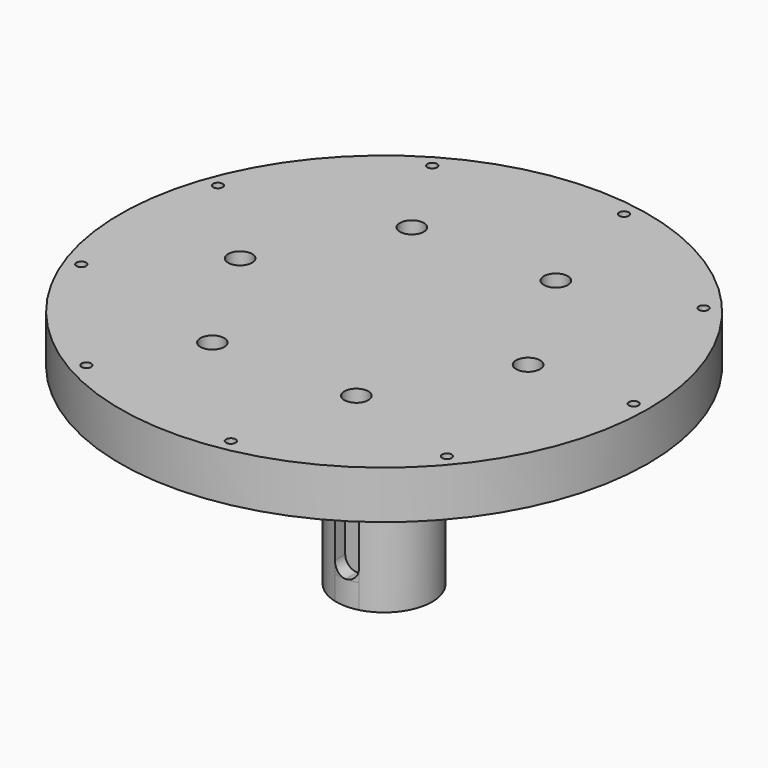
from build123d import *

# Parameters (mm, degrees)
F0_R         = 55
F0_R_2       = 1
F0_R_3       = 2.5
F0_R_4       = 10
F1_DEPTH     = 50
F1_FACE_R    = 55
F1_FACE_R_2  = 1
F1_FACE_R_3  = 2.5
F2_DEPTH     = 40
F3_R         = 7.5
F3_R_2       = 2.5
F4_DEPTH     = 5
F6_DEPTH     = 25
F7_DEPTH     = 5
F8_T4_DEPTH  = 15.1824583655
F8_S5_R      = 10
F8_T6_DEPTH  = 9
F8_T10_DEPTH = 15.1824583655
F8_S11_R     = 10
F8_T12_DEPTH = 9
F8_T16_DEPTH = 15.1824583655
F8_S17_R     = 10
F8_T18_DEPTH = 9
F8_T22_DEPTH = 15.1824583655
F8_S23_R     = 10
F8_T24_DEPTH = 9


# Not quite as in the source:
# - a fillet or chamfer that OpenCascade refuses, or shapes differently, is made with other operations: its cross-section is extruded or revolved along the edge and cut away or added


with BuildPart() as f1:
    # F0 (on Top) → F1 (new body)
    with BuildSketch(Plane.XY):
        Circle(F0_R)
        with Locations((-26, -45.0333209968)):
            Circle(F0_R_2, mode=Mode.SUBTRACT)
        with Locations((-48.8640162809, -17.7850474529)):
            Circle(F0_R_2, mode=Mode.SUBTRACT)
        with Locations((-15, -25.9807621135)):
            Circle(F0_R_3, mode=Mode.SUBTRACT)
        with Locations((9.0297052387, -51.2100031566)):
            Circle(F0_R_2, mode=Mode.SUBTRACT)
        with Locations((39.8343110422, -33.4249557037)):
            Circle(F0_R_2, mode=Mode.SUBTRACT)
        with Locations((15, -25.9807621135)):
            Circle(F0_R_3, mode=Mode.SUBTRACT)
        with Locations((-30, 0)):
            Circle(F0_R_3, mode=Mode.SUBTRACT)
        with Locations((-48.8640162809, 17.7850474529)):
            Circle(F0_R_2, mode=Mode.SUBTRACT)
        with Locations((-15, 25.9807621135)):
            Circle(F0_R_3, mode=Mode.SUBTRACT)
        with Locations((-26, 45.0333209968)):
            Circle(F0_R_2, mode=Mode.SUBTRACT)
        Circle(F0_R_4, mode=Mode.SUBTRACT)
        with Locations((15, 25.9807621135)):
            Circle(F0_R_3, mode=Mode.SUBTRACT)
        with Locations((30, 0)):
            Circle(F0_R_3, mode=Mode.SUBTRACT)
        with Locations((52, 0)):
            Circle(F0_R_2, mode=Mode.SUBTRACT)
        with Locations((9.0297052387, 51.2100031566)):
            Circle(F0_R_2, mode=Mode.SUBTRACT)
        with Locations((39.8343110422, 33.4249557037)):
            Circle(F0_R_2, mode=Mode.SUBTRACT)
        Circle(F0_R_4)
    extrude(amount=F1_DEPTH)

    # F0 (on Top) + F1_face (on face) → F2 (cut)
    with BuildSketch(Plane.XY):
        Circle(F0_R)
        with Locations((-26, -45.0333209968)):
            Circle(F0_R_2, mode=Mode.SUBTRACT)
        with Locations((-48.8640162809, -17.7850474529)):
            Circle(F0_R_2, mode=Mode.SUBTRACT)
        with Locations((-15, -25.9807621135)):
            Circle(F0_R_3, mode=Mode.SUBTRACT)
        with Locations((9.0297052387, -51.2100031566)):
            Circle(F0_R_2, mode=Mode.SUBTRACT)
        with Locations((39.8343110422, -33.4249557037)):
            Circle(F0_R_2, mode=Mode.SUBTRACT)
        with Locations((15, -25.9807621135)):
            Circle(F0_R_3, mode=Mode.SUBTRACT)
        with Locations((-30, 0)):
            Circle(F0_R_3, mode=Mode.SUBTRACT)
        with Locations((-48.8640162809, 17.7850474529)):
            Circle(F0_R_2, mode=Mode.SUBTRACT)
        with Locations((-15, 25.9807621135)):
            Circle(F0_R_3, mode=Mode.SUBTRACT)
        with Locations((-26, 45.0333209968)):
            Circle(F0_R_2, mode=Mode.SUBTRACT)
        Circle(F0_R_4, mode=Mode.SUBTRACT)
        with Locations((15, 25.9807621135)):
            Circle(F0_R_3, mode=Mode.SUBTRACT)
        with Locations((30, 0)):
            Circle(F0_R_3, mode=Mode.SUBTRACT)
        with Locations((52, 0)):
            Circle(F0_R_2, mode=Mode.SUBTRACT)
        with Locations((9.0297052387, 51.2100031566)):
            Circle(F0_R_2, mode=Mode.SUBTRACT)
        with Locations((39.8343110422, 33.4249557037)):
            Circle(F0_R_2, mode=Mode.SUBTRACT)
    with BuildSketch(Plane.XY.offset(50)):
        Circle(F1_FACE_R)
        with Locations((-26, -45.0333209968)):
            Circle(F1_FACE_R_2, mode=Mode.SUBTRACT)
        with Locations((-48.8640162809, -17.7850474529)):
            Circle(F1_FACE_R_2, mode=Mode.SUBTRACT)
        with Locations((-15, -25.9807621135)):
            Circle(F1_FACE_R_3, mode=Mode.SUBTRACT)
        with Locations((9.0297052387, -51.2100031566)):
            Circle(F1_FACE_R_2, mode=Mode.SUBTRACT)
        with Locations((39.8343110422, -33.4249557037)):
            Circle(F1_FACE_R_2, mode=Mode.SUBTRACT)
        with Locations((15, -25.9807621135)):
            Circle(F1_FACE_R_3, mode=Mode.SUBTRACT)
        with Locations((-30, 0)):
            Circle(F1_FACE_R_3, mode=Mode.SUBTRACT)
        with Locations((-48.8640162809, 17.7850474529)):
            Circle(F1_FACE_R_2, mode=Mode.SUBTRACT)
        with Locations((-15, 25.9807621135)):
            Circle(F1_FACE_R_3, mode=Mode.SUBTRACT)
        with Locations((-26, 45.0333209968)):
            Circle(F1_FACE_R_2, mode=Mode.SUBTRACT)
        with Locations((15, 25.9807621135)):
            Circle(F1_FACE_R_3, mode=Mode.SUBTRACT)
        with Locations((30, 0)):
            Circle(F1_FACE_R_3, mode=Mode.SUBTRACT)
        with Locations((52, 0)):
            Circle(F1_FACE_R_2, mode=Mode.SUBTRACT)
        with Locations((9.0297052387, 51.2100031566)):
            Circle(F1_FACE_R_2, mode=Mode.SUBTRACT)
        with Locations((39.8343110422, 33.4249557037)):
            Circle(F1_FACE_R_2, mode=Mode.SUBTRACT)
    extrude(amount=F2_DEPTH, mode=Mode.SUBTRACT)

    # F3 (on face) → F4 (cut)
    with BuildSketch(Plane(origin=(0, 0, 40), x_dir=(1, 0, 0), z_dir=(0, 0, -1))):
        with Locations((15, -25.9807621135)):
            Circle(F3_R)
        with Locations((15, -25.9807621135)):
            Circle(F3_R_2, mode=Mode.SUBTRACT)
        with Locations((30, 0)):
            Circle(F3_R)
        with Locations((30, 0)):
            Circle(F3_R_2, mode=Mode.SUBTRACT)
        with Locations((-15, -25.9807621135)):
            Circle(F3_R)
        with Locations((-15, -25.9807621135)):
            Circle(F3_R_2, mode=Mode.SUBTRACT)
        with Locations((15, 25.9807621135)):
            Circle(F3_R)
        with Locations((15, 25.9807621135)):
            Circle(F3_R_2, mode=Mode.SUBTRACT)
        with Locations((-15, 25.9807621135)):
            Circle(F3_R)
        with Locations((-15, 25.9807621135)):
            Circle(F3_R_2, mode=Mode.SUBTRACT)
        with Locations((-30, 0)):
            Circle(F3_R)
        with Locations((-30, 0)):
            Circle(F3_R_2, mode=Mode.SUBTRACT)
    extrude(amount=-F4_DEPTH, mode=Mode.SUBTRACT)

    # F5 (on face) → F6 (cut)
    with BuildSketch(Plane(origin=(0, 0, 0), x_dir=(1, 0, 0), z_dir=(0, 0, -1))):
        with BuildLine():
            Line((-2.5, 7), (0, 7))
            Line((0, 7), (2.5, 7))
            Line((2.5, 7), (2.5, 9.6824583655))
            ThreePointArc((2.5, 9.6824583655), (0, 10), (-2.5, 9.6824583655))
            Line((-2.5, 9.6824583655), (-2.5, 7))
        make_face()
    extrude(amount=-F6_DEPTH, mode=Mode.SUBTRACT)

    # F5 (on face) → F7 (join)
    with BuildSketch(Plane(origin=(0, 0, 0), x_dir=(1, 0, 0), z_dir=(0, 0, -1))):
        with BuildLine():
            Line((-2.5, 7), (0, 7))
            Line((0, 7), (2.5, 7))
            Line((2.5, 7), (2.5, 9.6824583655))
            ThreePointArc((2.5, 9.6824583655), (0, 10), (-2.5, 9.6824583655))
            Line((-2.5, 9.6824583655), (-2.5, 7))
        make_face()
    extrude(amount=-F7_DEPTH)

    # F8: fillet of radius 2.5 on 4 edges, made by hand


with BuildPart() as f8_tool2:
    # F8_s3 → F8_t4 (new body)
    with BuildSketch(Plane.XZ.offset(15.9324583655)):
        with BuildLine():
            ThreePointArc((-2.5, 22.5), (-1.767766953, 24.267766953), (0, 25))
            Line((0, 25), (-2.5, 25))
            Line((-2.5, 25), (-2.5, 22.5))
        make_face()
    extrude(amount=-F8_T4_DEPTH)

    # F8_s5 → F8_t6 (intersect, symmetric)
    with BuildSketch(Plane.XY.offset(23.8)):
        Circle(F8_S5_R)
    extrude(amount=F8_T6_DEPTH, both=True, mode=Mode.INTERSECT)


with BuildPart() as f1_1:
    add(f1.part)

    # F8_t1: union F8_tool2
    add(f8_tool2.part)


with BuildPart() as f8_tool8:
    # F8_s9 → F8_t10 (new body)
    with BuildSketch(Plane.XZ.offset(0.75)):
        with BuildLine():
            ThreePointArc((0, 25), (1.767766953, 24.267766953), (2.5, 22.5))
            Line((2.5, 22.5), (2.5, 25))
            Line((2.5, 25), (0, 25))
        make_face()
    extrude(amount=F8_T10_DEPTH)

    # F8_s11 → F8_t12 (intersect, symmetric)
    with BuildSketch(Plane.XY.offset(23.8)):
        Circle(F8_S11_R)
    extrude(amount=F8_T12_DEPTH, both=True, mode=Mode.INTERSECT)


with BuildPart() as f1_2:
    add(f1_1.part)

    # F8_t7: union F8_tool8
    add(f8_tool8.part)


with BuildPart() as f8_tool14:
    # F8_s15 → F8_t16 (new body)
    with BuildSketch(Plane.XZ.offset(0.75)):
        with BuildLine():
            ThreePointArc((2.5, 7.5), (1.767766953, 5.732233047), (0, 5))
            Line((0, 5), (2.5, 5))
            Line((2.5, 5), (2.5, 7.5))
        make_face()
    extrude(amount=F8_T16_DEPTH)

    # F8_s17 → F8_t18 (intersect, symmetric)
    with BuildSketch(Plane.XY.offset(6.2)):
        Circle(F8_S17_R)
    extrude(amount=F8_T18_DEPTH, both=True, mode=Mode.INTERSECT)


with BuildPart() as f1_3:
    add(f1_2.part)

    # F8_t13: union F8_tool14
    add(f8_tool14.part)


with BuildPart() as f8_tool20:
    # F8_s21 → F8_t22 (new body)
    with BuildSketch(Plane.XZ.offset(15.9324583655)):
        with BuildLine():
            ThreePointArc((-2.5, 7.5), (-1.767766953, 5.732233047), (0, 5))
            Line((0, 5), (-2.5, 5))
            Line((-2.5, 5), (-2.5, 7.5))
        make_face()
    extrude(amount=-F8_T22_DEPTH)

    # F8_s23 → F8_t24 (intersect, symmetric)
    with BuildSketch(Plane.XY.offset(6.2)):
        Circle(F8_S23_R)
    extrude(amount=F8_T24_DEPTH, both=True, mode=Mode.INTERSECT)


with BuildPart() as f1_4:
    add(f1_3.part)

    # F8_t19: union F8_tool20
    add(f8_tool20.part)


solid = f1_4.part
